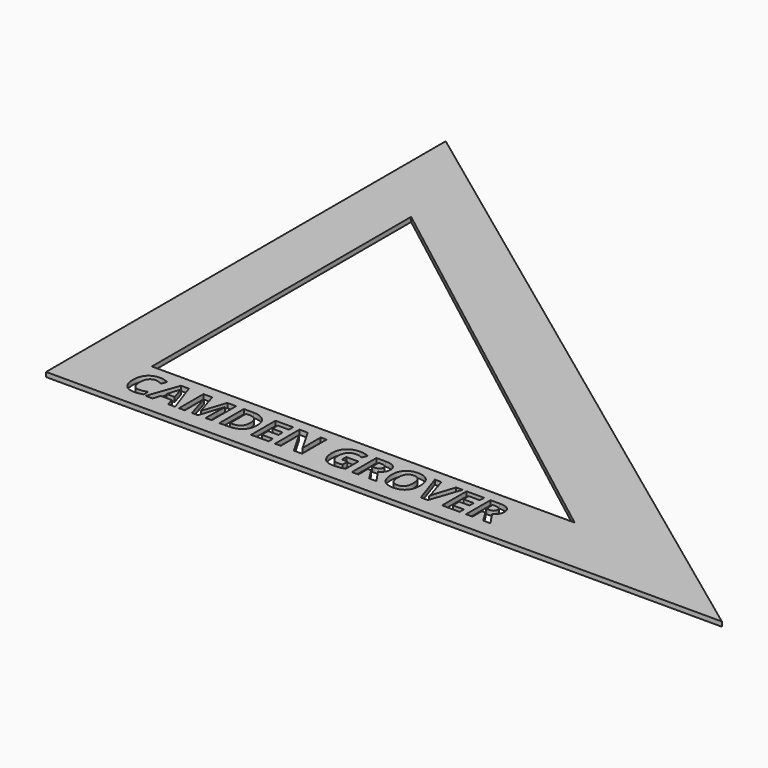
from build123d import *

# Parameters (mm, degrees)
F1_DEPTH     = 2
F2_SCALE     = 0.75
F3_TEXT_SIZE = 13.8751121122
F4_DEPTH     = 1.501


# Not quite as in the source:
# - Text() gives the source's letters only with a copy of the font that has no kerning and outlines rounded to 1/6400 em; it was checked with that copy


with BuildPart() as f1:
    # F0 (on Top) → F1 (new body)
    with BuildSketch(Plane.XY):
        Polygon((-110.3935540405, 109.5033976257), (-110.3935540405, -106.3966023743), (181.7064459595, -106.3966023743), align=None)
        Polygon((-84.9935540405, -80.9966023743), (-84.9935540405, 59.0477188125), (97.7188157638, -80.9966023743), align=None, mode=Mode.SUBTRACT)
    extrude(amount=F1_DEPTH)


with BuildPart() as f1_1:
    # F2: moved
    add(f1.part.scale(F2_SCALE))

    # F3 (on face) → F4 (cut, through all)
    with BuildSketch(Plane.XY.offset(1.5)):
        with Locations((-63.7451655304, -74.3297189474)):
            Text('CAMDEN GROVER', F3_TEXT_SIZE, font='Open Sans', font_style=FontStyle.BOLD, text_align=(TextAlign.LEFT, TextAlign.BOTTOM))
    extrude(amount=-F4_DEPTH, mode=Mode.SUBTRACT)


solid = f1_1.part
